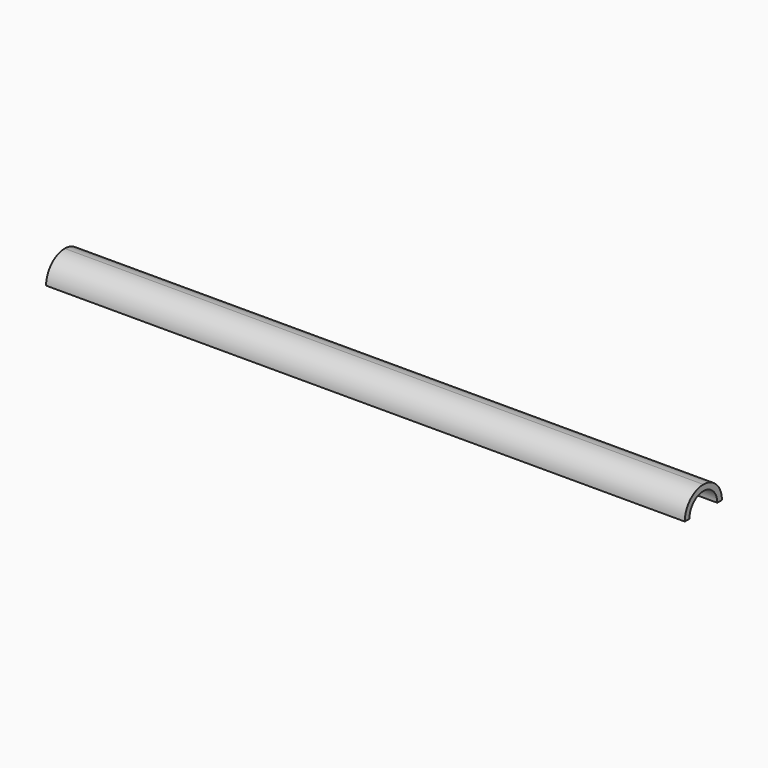
from build123d import *

# Parameters (mm, degrees)
F0_W     = 69.85
F0_H     = 5.08
F1_DEPTH = 2.54
F2_R     = 2.53999
F4_D     = 3.81


# Not quite as in the source:
# - a fillet or chamfer is up to 0.001 mm smaller than in the source, because OpenCascade refuses the exact size


with BuildPart() as f1:
    # F0 (on Top) → F1 (new body)
    with BuildSketch(Plane.XY):
        with Locations((-40.0687940419, 48.9344280766)):
            Rectangle(F0_W, F0_H)
    extrude(amount=F1_DEPTH)

    # F2 (radius 2.54 in the source; OpenCascade refuses exactly that, so slightly less here)
    f2_edges = [f1.edges().sort_by_distance(p)[0] for p in [
        (-40.068794, 46.394428, 2.54),
        (-40.068794, 51.474428, 2.54),
    ]]
    fillet(f2_edges, radius=F2_R)

    # F4 (through all)
    with Locations(Plane.YZ.offset(-5.1437940419)):
        with Locations((48.9344280766, 0)):
            Hole(F4_D / 2)


solid = f1.part
